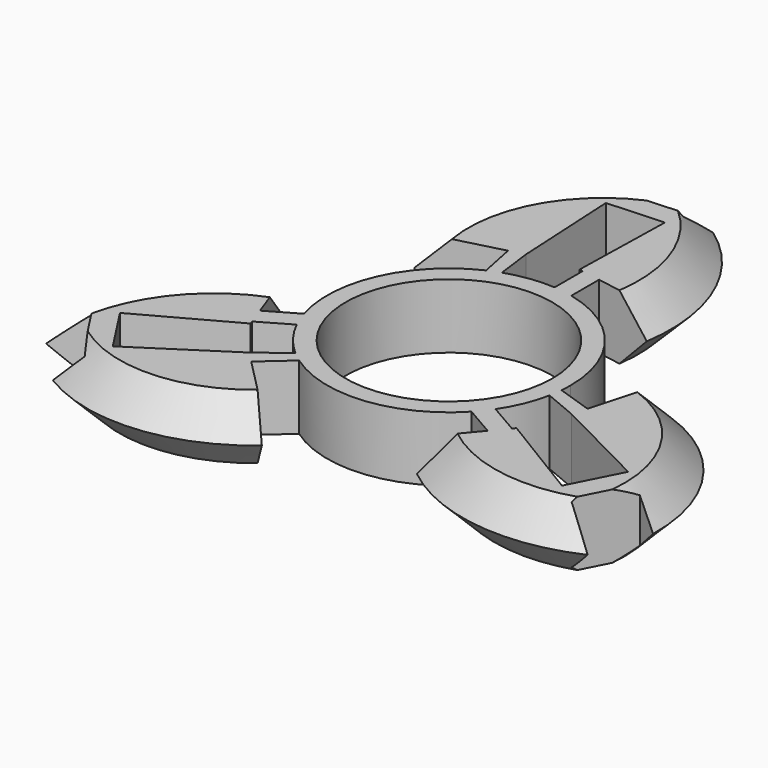
from build123d import *

# Parameters (mm, degrees)
F0_R     = 11.2
F1_DEPTH = 7
F2_SIZE  = 3.5
F3_SIZE  = 3.49999


# Not quite as in the source:
# - a fillet or chamfer is up to 0.001 mm smaller than in the source, because OpenCascade refuses the exact size


with BuildPart() as f1:
    # F0 (on Top) → F1 (new body)
    with BuildSketch(Plane.XY):
        Polygon((-5.4887417888, 30.3404310419), (-5.3626246511, 27.9541106613), (0.7814850479, 28.2788271306), (0.8367048606, 30.6747311771), align=None)
        with BuildLine():
            Line((-6.3603435788, 15.9527909689), (-4.7504720739, 16.3712901342))
            Line((-4.7504720739, 16.3712901342), (-5.3626246511, 27.9541106613))
            Line((-5.3626246511, 27.9541106613), (-5.4887417888, 30.3404310419))
            Line((-5.4887417888, 30.3404310419), (-5.6316571191, 33.0445977541))
            ThreePointArc((-5.6316571191, 33.0445977541), (-13.3586462682, 24.898567552), (-14.7876461409, 13.7620452616))
            Line((-14.7876461409, 13.7620452616), (-6.3603435788, 15.9527909689))
        make_face()
        with BuildLine():
            ThreePointArc((-5.5532608378, 11.975027936), (-4.9107856444, 12.2525174701), (-4.2545066222, 12.4955661497))
            Line((-4.2545066222, 12.4955661497), (-4.7504720739, 16.3712901342))
            Line((-4.7504720739, 16.3712901342), (-6.3603435788, 15.9527909689))
            Line((-6.3603435788, 15.9527909689), (-5.5532608378, 11.975027936))
        make_face()
        with BuildLine():
            Line((0.912733085, 16.988074322), (2.9751978168, 16.625185455))
            Line((2.9751978168, 16.625185455), (8.9877722785, 15.5672782332))
            ThreePointArc((8.9877722785, 15.5672782332), (7.6544413443, 26.2358342161), (0.9277061572, 34.6231396156))
            Line((0.9277061572, 34.6231396156), (0.8367048606, 30.6747311771))
            Line((0.8367048606, 30.6747311771), (0.7814850479, 28.2788271306))
            Line((0.7814850479, 28.2788271306), (0.5228415025, 17.0566754052))
            Line((0.5228415025, 17.0566754052), (0.912733085, 16.988074322))
        make_face()
        with BuildLine():
            ThreePointArc((0.912733085, 13.1684060659), (1.9500586477, 13.055162629), (2.9751978168, 12.8603342861))
            Line((2.9751978168, 12.8603342861), (2.9751978168, 16.625185455))
            Line((2.9751978168, 16.625185455), (0.912733085, 16.988074322))
            Line((0.912733085, 16.988074322), (0.912733085, 13.1684060659))
        make_face()
        with BuildLine():
            ThreePointArc((13.1473088225, -1.1782490086), (13.1868206262, -0.5897132961), (13.2, 0))
            ThreePointArc((13.2, 0), (10.3322943043, 8.214845976), (2.9751978168, 12.8603342861))
            ThreePointArc((2.9751978168, 12.8603342861), (1.9500586477, 13.055162629), (0.912733085, 13.1684060659))
            ThreePointArc((0.912733085, 13.1684060659), (-1.7044180771, 13.089498043), (-4.2545066222, 12.4955661497))
            ThreePointArc((-4.2545066222, 12.4955661497), (-4.9107856444, 12.2525174701), (-5.5532608378, 11.975027936))
            ThreePointArc((-5.5532608378, 11.975027936), (-12.0518959346, 5.3844038094), (-12.6249751013, -3.8535702524))
            ThreePointArc((-12.6249751013, -3.8535702524), (-12.2811318111, -4.8387809867), (-11.8605407229, -5.7937529945))
            ThreePointArc((-11.8605407229, -5.7937529945), (-10.4836287895, -8.020818375), (-8.6942244092, -9.9322938902))
            ThreePointArc((-8.6942244092, -9.9322938902), (-8.1555985672, -10.3791238557), (-7.5940479846, -10.7967789274))
            ThreePointArc((-7.5940479846, -10.7967789274), (1.3629174841, -13.1294499478), (9.6497772845, -9.0067640337))
            ThreePointArc((9.6497772845, -9.0067640337), (10.3310731634, -8.2163816423), (10.9478076379, -7.3746530714))
            ThreePointArc((10.9478076379, -7.3746530714), (12.1880468666, -5.068679668), (12.9487310314, -2.5632722595))
            ThreePointArc((12.9487310314, -2.5632722595), (13.0663842116, -1.8733936144), (13.1473088225, -1.1782490086))
        make_face()
        Circle(F0_R, mode=Mode.SUBTRACT)
        with BuildLine():
            Line((-15.1684704667, -7.7035871225), (-15.885431855, -5.7359958369))
            Line((-15.885431855, -5.7359958369), (-17.975544557, 0))
            ThreePointArc((-17.975544557, 0), (-26.5481195928, -6.4889764521), (-30.4483715445, -16.5081527084))
            Line((-30.4483715445, -16.5081527084), (-26.983448884, -14.6127579238))
            Line((-26.983448884, -14.6127579238), (-24.8809252083, -13.4626276612))
            Line((-24.8809252083, -13.4626276612), (-15.0329349563, -8.0755436793))
            Line((-15.0329349563, -8.0755436793), (-15.1684704667, -7.7035871225))
        make_face()
        with BuildLine():
            ThreePointArc((-11.8605407229, -5.7937529945), (-12.2811318111, -4.8387809867), (-12.6249751013, -3.8535702524))
            Line((-12.6249751013, -3.8535702524), (-15.885431855, -5.7359958369))
            Line((-15.885431855, -5.7359958369), (-15.1684704667, -7.7035871225))
            Line((-15.1684704667, -7.7035871225), (-11.8605407229, -5.7937529945))
        make_face()
        with BuildLine():
            Line((-10.6353504509, -13.4846146005), (-7.5940479846, -10.7967789274))
            ThreePointArc((-7.5940479846, -10.7967789274), (-8.1555985672, -10.3791238557), (-8.6942244092, -9.9322938902))
            Line((-8.6942244092, -9.9322938902), (-11.802717112, -12.2996745631))
            Line((-11.802717112, -12.2996745631), (-10.6353504509, -13.4846146005))
        make_face()
        with BuildLine():
            Line((-4.5244577341, -19.687499851), (-10.6353504509, -13.4846146005))
            Line((-10.6353504509, -13.4846146005), (-11.802717112, -12.2996745631))
            Line((-11.802717112, -12.2996745631), (-21.5276576473, -18.6212245095))
            Line((-21.5276576473, -18.6212245095), (-23.5312131497, -19.9236053449))
            Line((-23.5312131497, -19.9236053449), (-25.8016325533, -21.3994570076))
            ThreePointArc((-25.8016325533, -21.3994570076), (-14.8834688838, -24.0182108044), (-4.5244577341, -19.687499851))
        make_face()
        Polygon((-23.5312131497, -19.9236053449), (-21.5276576473, -18.6212245095), (-24.8809252083, -13.4626276612), (-26.983448884, -14.6127579238), align=None)
        with BuildLine():
            Line((14.2557373817, -9.2844871995), (10.9478076379, -7.3746530714))
            ThreePointArc((10.9478076379, -7.3746530714), (10.3310731634, -8.2163816423), (9.6497772845, -9.0067640337))
            Line((9.6497772845, -9.0067640337), (12.9102340382, -10.8891896181))
            Line((12.9102340382, -10.8891896181), (14.2557373817, -9.2844871995))
        make_face()
        with BuildLine():
            Line((14.5100934538, -8.9811317259), (14.2557373817, -9.2844871995))
            Line((14.2557373817, -9.2844871995), (12.9102340382, -10.8891896181))
            Line((12.9102340382, -10.8891896181), (8.9877722785, -15.5672782332))
            ThreePointArc((8.9877722785, -15.5672782332), (18.8936782485, -19.746857764), (29.5206653873, -18.1149869072))
            Line((29.5206653873, -18.1149869072), (26.1467440233, -16.0619732533))
            Line((26.1467440233, -16.0619732533), (24.0994401604, -14.8161994695))
            Line((24.0994401604, -14.8161994695), (14.5100934538, -8.9811317259))
        make_face()
        Polygon((29.0199549385, -10.416825697), (26.8902822984, -9.3328861518), (24.0994401604, -14.8161994695), (26.1467440233, -16.0619732533), align=None)
        with BuildLine():
            Line((19.312103875, 5.9254545894), (16.9956940297, -2.4681763684))
            Line((16.9956940297, -2.4681763684), (16.5531891859, -4.0716155711))
            Line((16.5531891859, -4.0716155711), (26.8902822984, -9.3328861518))
            Line((26.8902822984, -9.3328861518), (29.0199549385, -10.416825697))
            Line((29.0199549385, -10.416825697), (31.4332896725, -11.6451407465))
            ThreePointArc((31.4332896725, -11.6451407465), (28.242115152, -0.8803567476), (19.312103875, 5.9254545894))
        make_face()
        with BuildLine():
            Line((16.9956940297, -2.4681763684), (13.1473088225, -1.1782490086))
            ThreePointArc((13.1473088225, -1.1782490086), (13.0663842116, -1.8733936144), (12.9487310314, -2.5632722595))
            Line((12.9487310314, -2.5632722595), (16.5531891859, -4.0716155711))
            Line((16.5531891859, -4.0716155711), (16.9956940297, -2.4681763684))
        make_face()
    extrude(amount=F1_DEPTH)

    # F2
    f2_edges = [f1.edges().sort_by_distance(p)[0] for p in [
        (-13.358646, 24.898568, 7),
        (7.654441, 26.235834, 7),
        (28.242115, -0.880357, 7),
        (18.893678, -19.746858, 7),
        (-14.883469, -24.018211, 7),
        (-26.54812, -6.488976, 7),
    ]]
    chamfer(f2_edges, length=F2_SIZE)

    # F3 (size 3.5 in the source; OpenCascade refuses exactly that, so slightly less here)
    f3_edges = [f1.edges().sort_by_distance(p)[0] for p in [
        (7.654441, 26.235834, 0),
        (-13.358646, 24.898568, 0),
        (-26.54812, -6.488976, 0),
        (-14.883469, -24.018211, 0),
        (18.893678, -19.746858, 0),
        (28.242115, -0.880357, 0),
    ]]
    chamfer(f3_edges, length=F3_SIZE)


solid = f1.part
